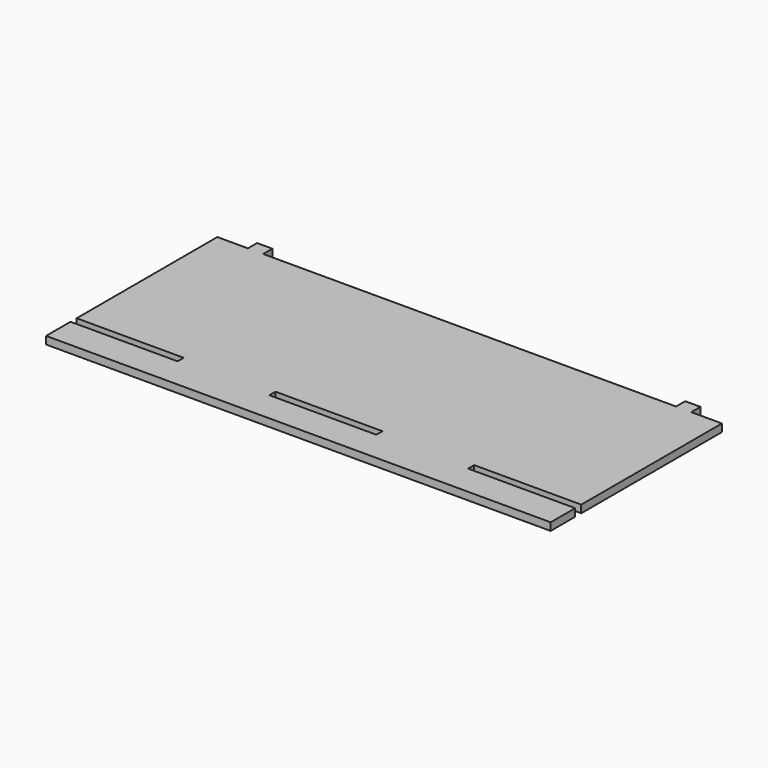
from build123d import *

# Parameters (mm, degrees)
F0_W     = 209.55
F0_H     = 88.9
F1_DEPTH = 3.175
F2_W     = 44.45
F2_H     = 3.175
F3_DEPTH = 25.4
F4_W     = 6.35
F4_H     = 4.7625
F5_DEPTH = 3.175


# Not quite as in the source:
# - a length typed as a fraction of an inch, garbled in the dataset ("3 / 203.2 mm" for 3/8 in), is restored


with BuildPart() as f1:
    # F0 (on Top) → F1 (new body)
    with BuildSketch(Plane.XY):
        Rectangle(F0_W, F0_H)
    extrude(amount=F1_DEPTH)

    # F2 (on face) → F3 (cut)
    with BuildSketch(Plane.XY.offset(3.175)):
        with Locations((-82.55, -30.1625)):
            Rectangle(F2_W, F2_H)
        with Locations((82.55, -30.1625)):
            Rectangle(F2_W, F2_H)
        with Locations((0, -30.1625)):
            Rectangle(F2_W, F2_H)
    extrude(amount=-F3_DEPTH, mode=Mode.SUBTRACT)

    # F4 (on face) → F5 (join)
    with BuildSketch(Plane.XY.offset(3.175)):
        with Locations((-88.9, 46.83125)):
            Rectangle(F4_W, F4_H)
        with Locations((88.9, 46.83125)):
            Rectangle(F4_W, F4_H)
    extrude(amount=-F5_DEPTH)


solid = f1.part
